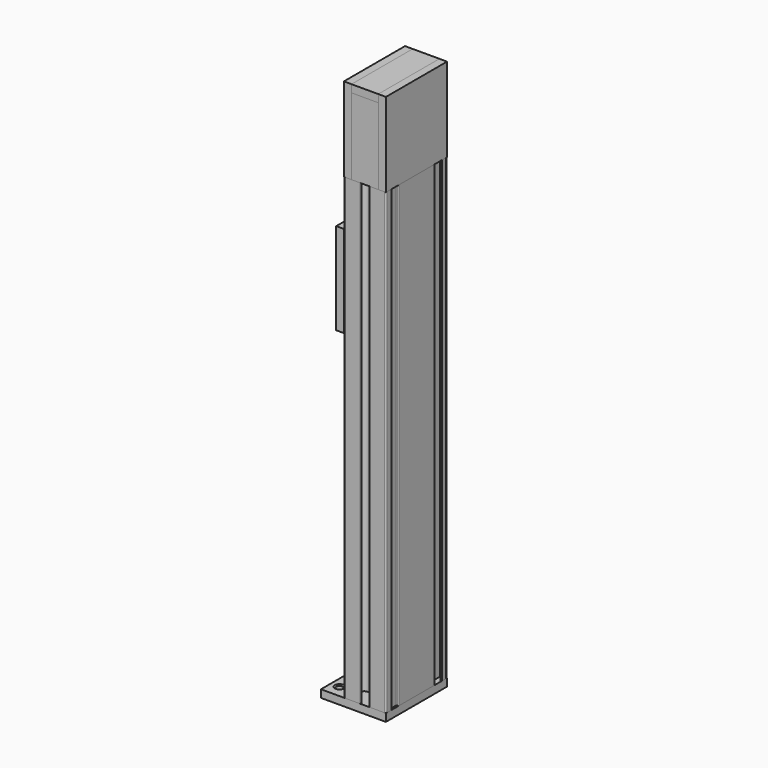
from build123d import *

# Parameters (mm, degrees)
F1_DEPTH        = 600
F2_W            = 100
F2_H            = 110
F3_DEPTH        = 10
F4_W            = 100
F4_H            = 110
F5_DEPTH        = 10
F6_W            = 100
F6_H            = 10
F7_DEPTH        = 35
F8_W            = 35
F8_H            = 100
F9_DEPTH        = 10
F10_W           = 35
F10_H           = 100
F11_DEPTH       = 10
F12_W           = 85
F12_H           = 100
F13_DEPTH       = 10
F15_D           = 9
F15_CSINK_D     = 12
F15_CSINK_ANGLE = 90
F16_W           = 100
F16_H           = 120
F17_DEPTH       = 10
F19_D           = 9
F19_CSINK_D     = 11
F19_CSINK_ANGLE = 90
F21_DEPTH       = 65.001


with BuildPart() as f1:
    # F0 (on Top) → F1 (new body)
    with BuildSketch(Plane.XY):
        with BuildLine():
            Line((8.33733906, -48), (6.5, -48))
            ThreePointArc((6.5, -48), (5.5, -49), (6.5, -50))
            Line((6.5, -50), (25.5, -50))
            ThreePointArc((25.5, -50), (26.9142135624, -49.4142135624), (27.5, -48))
            Line((27.5, -48), (27.5, -41.5))
            ThreePointArc((27.5, -41.5), (27.2071067812, -40.7928932188), (26.5, -40.5))
            Line((26.5, -40.5), (25.30947502, -40.5))
            ThreePointArc((25.30947502, -40.5), (24.9559216294, -40.3535533906), (24.80947502, -40))
            Line((24.80947502, -40), (24.80947502, -30))
            ThreePointArc((24.80947502, -30), (24.9559216294, -29.6464466094), (25.30947502, -29.5))
            Line((25.30947502, -29.5), (26.5, -29.5))
            ThreePointArc((26.5, -29.5), (27.2071067812, -29.2071067812), (27.5, -28.5))
            Line((27.5, -28.5), (27.5, 29))
            ThreePointArc((27.5, 29), (26.5, 30), (25.5, 29))
            Line((25.5, 29), (25.5, 24))
            ThreePointArc((25.5, 24), (25.3535533906, 23.6464466094), (25, 23.5))
            Line((25, 23.5), (20.5, 23.5))
            ThreePointArc((20.5, 23.5), (20.1464466094, 23.6464466094), (20, 24))
            Line((20, 24), (20, 47.5))
            ThreePointArc((20, 47.5), (20.1464466094, 47.8535533906), (20.5, 48))
            Line((20.5, 48), (25, 48))
            ThreePointArc((25, 48), (25.3535533906, 47.8535533906), (25.5, 47.5))
            Line((25.5, 47.5), (25.5, 42))
            ThreePointArc((25.5, 42), (26.5, 41), (27.5, 42))
            Line((27.5, 42), (27.5, 48))
            ThreePointArc((27.5, 48), (26.9142135624, 49.4142135624), (25.5, 50))
            Line((25.5, 50), (7, 50))
            ThreePointArc((7, 50), (6, 49), (7, 48))
            Line((7, 48), (17.5, 48))
            ThreePointArc((17.5, 48), (17.8535533906, 47.8535533906), (18, 47.5))
            Line((18, 47.5), (18, 40.5))
            ThreePointArc((18, 40.5), (17.8535533906, 40.1464466094), (17.5, 40))
            Line((17.5, 40), (-17.5, 40))
            ThreePointArc((-17.5, 40), (-17.8535533906, 40.1464466094), (-18, 40.5))
            Line((-18, 40.5), (-18, 47.5))
            ThreePointArc((-18, 47.5), (-17.8535533906, 47.8535533906), (-17.5, 48))
            Line((-17.5, 48), (-7, 48))
            ThreePointArc((-7, 48), (-6, 49), (-7, 50))
            Line((-7, 50), (-25.5, 50))
            ThreePointArc((-25.5, 50), (-26.9142135624, 49.4142135624), (-27.5, 48))
            Line((-27.5, 48), (-27.5, 42))
            ThreePointArc((-27.5, 42), (-26.5, 41), (-25.5, 42))
            Line((-25.5, 42), (-25.5, 47.5))
            ThreePointArc((-25.5, 47.5), (-25.3535533906, 47.8535533906), (-25, 48))
            Line((-25, 48), (-20.5, 48))
            ThreePointArc((-20.5, 48), (-20.1464466094, 47.8535533906), (-20, 47.5))
            Line((-20, 47.5), (-20, 24))
            ThreePointArc((-20, 24), (-20.1464466094, 23.6464466094), (-20.5, 23.5))
            Line((-20.5, 23.5), (-25, 23.5))
            ThreePointArc((-25, 23.5), (-25.3535533906, 23.6464466094), (-25.5, 24))
            Line((-25.5, 24), (-25.5, 29))
            ThreePointArc((-25.5, 29), (-26.5, 30), (-27.5, 29))
            Line((-27.5, 29), (-27.5, -28.5))
            ThreePointArc((-27.5, -28.5), (-27.2071067812, -29.2071067812), (-26.5, -29.5))
            Line((-26.5, -29.5), (-25.30947502, -29.5))
            ThreePointArc((-25.30947502, -29.5), (-24.9559216294, -29.6464466094), (-24.80947502, -30))
            Line((-24.80947502, -30), (-24.80947502, -40))
            ThreePointArc((-24.80947502, -40), (-24.9559216294, -40.3535533906), (-25.30947502, -40.5))
            Line((-25.30947502, -40.5), (-26.5, -40.5))
            ThreePointArc((-26.5, -40.5), (-27.2071067812, -40.7928932188), (-27.5, -41.5))
            Line((-27.5, -41.5), (-27.5, -48))
            ThreePointArc((-27.5, -48), (-26.9142135624, -49.4142135624), (-25.5, -50))
            Line((-25.5, -50), (-6.5, -50))
            ThreePointArc((-6.5, -50), (-5.5, -49), (-6.5, -48))
            Line((-6.5, -48), (-8.33733906, -48))
            ThreePointArc((-8.33733906, -48), (-8.6908924506, -47.8535533906), (-8.83733906, -47.5))
            Line((-8.83733906, -47.5), (-8.83733906, -46))
            ThreePointArc((-8.83733906, -46), (-8.9837856694, -45.6464466094), (-9.33733906, -45.5))
            Line((-9.33733906, -45.5), (-11.8095842402, -45.5))
            ThreePointArc((-11.8095842402, -45.5), (-12.0057003753, -45.5400668945), (-12.1703854525, -45.6538461538))
            ThreePointArc((-12.1703854525, -45.6538461538), (-17.9864641346, -47.3129531545), (-22.2921545673, -43.0655495741))
            ThreePointArc((-22.2921545673, -43.0655495741), (-22.3051259928, -43.0008907051), (-22.30947502, -42.9350871095))
            Line((-22.30947502, -42.9350871095), (-22.30947502, -29.0649128904))
            ThreePointArc((-22.30947502, -29.0649128904), (-22.3051259928, -28.9991092949), (-22.2921545673, -28.934450426))
            ThreePointArc((-22.2921545673, -28.934450426), (-18.8105481092, -24.9627292431), (-13.5385137945, -25.2818011292))
            ThreePointArc((-13.5385137945, -25.2818011292), (-12.4221432577, -26.0444644798), (-11.0970213481, -26.3127749093))
            Line((-11.0970213481, -26.3127749093), (-9.33733906, -26.3127749093))
            ThreePointArc((-9.33733906, -26.3127749093), (-8.9837856694, -26.1663282999), (-8.83733906, -25.8127749093))
            Line((-8.83733906, -25.8127749093), (-8.83733906, -21.1))
            ThreePointArc((-8.83733906, -21.1), (-8.3687099099, -19.9686291501), (-7.23733906, -19.5))
            Line((-7.23733906, -19.5), (7.23733906, -19.5))
            ThreePointArc((7.23733906, -19.5), (8.3687099099, -19.9686291501), (8.83733906, -21.1))
            Line((8.83733906, -21.1), (8.83733906, -25.8127749093))
            ThreePointArc((8.83733906, -25.8127749093), (8.9837856694, -26.1663282999), (9.33733906, -26.3127749093))
            Line((9.33733906, -26.3127749093), (11.0970213482, -26.3127749093))
            ThreePointArc((11.0970213482, -26.3127749093), (12.4221432577, -26.0444644798), (13.5385137946, -25.2818011292))
            ThreePointArc((13.5385137946, -25.2818011292), (18.8105481092, -24.9627292431), (22.2921545673, -28.9344504259))
            ThreePointArc((22.2921545673, -28.9344504259), (22.3051259928, -28.9991092949), (22.30947502, -29.0649128904))
            Line((22.30947502, -29.0649128904), (22.30947502, -42.9350871095))
            ThreePointArc((22.30947502, -42.9350871095), (22.3051259928, -43.0008907051), (22.2921545673, -43.0655495741))
            ThreePointArc((22.2921545673, -43.0655495741), (17.9864641346, -47.3129531545), (12.1703854525, -45.6538461538))
            ThreePointArc((12.1703854525, -45.6538461538), (12.0057003753, -45.5400668945), (11.8095842402, -45.5))
            Line((11.8095842402, -45.5), (9.33733906, -45.5))
            ThreePointArc((9.33733906, -45.5), (8.9837856694, -45.6464466094), (8.83733906, -46))
            Line((8.83733906, -46), (8.83733906, -47.5))
            ThreePointArc((8.83733906, -47.5), (8.6908924506, -47.8535533906), (8.33733906, -48))
        make_face()
        with BuildLine():
            Line((25.5, 14.6098564162), (25.5, -14.1098564162))
            ThreePointArc((25.5, -14.1098564162), (25.2937023297, -14.5145031034), (24.8450442339, -14.5852391152))
            ThreePointArc((24.8450442339, -14.5852391152), (23.1777547131, -15.1146259293), (23.1458153918, -16.8636498356))
            ThreePointArc((23.1458153918, -16.8636498356), (21.5, -20), (19.8541846082, -16.8636498356))
            ThreePointArc((19.8541846082, -16.8636498356), (19.4720856876, -14.7770256685), (17.3854615204, -15.1591245891))
            ThreePointArc((17.3854615204, -15.1591245891), (16.5045669812, -18.2136561594), (17.6430539208, -21.1818181818))
            ThreePointArc((17.6430539208, -21.1818181818), (17.7096263297, -21.7132007164), (17.2573593129, -22))
            Line((17.2573593129, -22), (11.83733906, -22))
            ThreePointArc((11.83733906, -22), (11.4837856694, -21.8535533906), (11.33733906, -21.5))
            Line((11.33733906, -21.5), (11.33733906, -21.1))
            ThreePointArc((11.33733906, -21.1), (10.1364768629, -18.2008621971), (7.23733906, -17))
            Line((7.23733906, -17), (-7.23733906, -17))
            ThreePointArc((-7.23733906, -17), (-10.1364768629, -18.2008621971), (-11.33733906, -21.1))
            Line((-11.33733906, -21.1), (-11.33733906, -21.5))
            ThreePointArc((-11.33733906, -21.5), (-11.4837856694, -21.8535533906), (-11.83733906, -22))
            Line((-11.83733906, -22), (-17.2573593129, -22))
            ThreePointArc((-17.2573593129, -22), (-17.7096263297, -21.7132007164), (-17.6430539208, -21.1818181818))
            ThreePointArc((-17.6430539208, -21.1818181818), (-16.5045669812, -18.2136561594), (-17.3854615204, -15.1591245891))
            ThreePointArc((-17.3854615204, -15.1591245891), (-19.4720856876, -14.7770256685), (-19.8541846082, -16.8636498356))
            ThreePointArc((-19.8541846082, -16.8636498356), (-21.5, -20), (-23.1458153918, -16.8636498356))
            ThreePointArc((-23.1458153918, -16.8636498356), (-23.1777547131, -15.1146259293), (-24.8450442339, -14.5852391152))
            ThreePointArc((-24.8450442339, -14.5852391152), (-25.2937023297, -14.5145031034), (-25.5, -14.1098564162))
            Line((-25.5, -14.1098564162), (-25.5, 14.6098564162))
            ThreePointArc((-25.5, 14.6098564162), (-25.2937023297, 15.0145031034), (-24.8450442339, 15.0852391152))
            ThreePointArc((-24.8450442339, 15.0852391152), (-23.1777547131, 15.6146259293), (-23.1458153918, 17.3636498356))
            ThreePointArc((-23.1458153918, 17.3636498356), (-21.5, 20.5), (-19.8541846082, 17.3636498356))
            ThreePointArc((-19.8541846082, 17.3636498356), (-19.4720856876, 15.2770256685), (-17.3854615204, 15.6591245891))
            ThreePointArc((-17.3854615204, 15.6591245891), (-16.514462151, 18.8800162584), (-17.8635792315, 21.9316823854))
            ThreePointArc((-17.8635792315, 21.9316823854), (-17.9646454387, 22.0902903218), (-18, 22.2750087852))
            Line((-18, 22.2750087852), (-18, 36.5))
            ThreePointArc((-18, 36.5), (-17.7071067812, 37.2071067812), (-17, 37.5))
            Line((-17, 37.5), (17, 37.5))
            ThreePointArc((17, 37.5), (17.7071067812, 37.2071067812), (18, 36.5))
            Line((18, 36.5), (18, 22.2750087852))
            ThreePointArc((18, 22.2750087852), (17.9646454387, 22.0902903218), (17.8635792315, 21.9316823854))
            ThreePointArc((17.8635792315, 21.9316823854), (16.514462151, 18.8800162584), (17.3854615204, 15.6591245891))
            ThreePointArc((17.3854615204, 15.6591245891), (19.4720856876, 15.2770256685), (19.8541846082, 17.3636498356))
            ThreePointArc((19.8541846082, 17.3636498356), (19.6774992234, 19.3237056022), (21.2654667699, 20.4862009375))
            ThreePointArc((21.2654667699, 20.4862009375), (22.3229466011, 17.3003700971), (24.8450442339, 15.0852391152))
            ThreePointArc((24.8450442339, 15.0852391152), (25.2937023297, 15.0145031034), (25.5, 14.6098564162))
        make_face(mode=Mode.SUBTRACT)
    extrude(amount=-F1_DEPTH)


with BuildPart() as f3:
    # F2 (on face) → F3 (new body)
    with BuildSketch(Plane.YZ.offset(27.5)):
        with Locations((0, 55)):
            Rectangle(F2_W, F2_H)
    extrude(amount=-F3_DEPTH)


with BuildPart() as f5:
    # F4 (on face) → F5 (new body)
    with BuildSketch(Plane(origin=(-27.5, 0, 0), x_dir=(0, -1, 0), z_dir=(-1, 0, 0))):
        with Locations((0, 55)):
            Rectangle(F4_W, F4_H)
    extrude(amount=-F5_DEPTH)


with BuildPart() as f7:
    # F6 (on face) → F7 (new body, through all)
    with BuildSketch(Plane(origin=(17.5, 0, 0), x_dir=(0, -1, 0), z_dir=(-1, 0, 0))):
        with Locations((0, 105)):
            Rectangle(F6_W, F6_H)
    extrude(amount=F7_DEPTH)


with BuildPart() as f9:
    # F8 (on face) → F9 (new body)
    with BuildSketch(Plane.XZ.offset(50)):
        with Locations((0, 50)):
            Rectangle(F8_W, F8_H)
    extrude(amount=-F9_DEPTH)


with BuildPart() as f11:
    # F10 (on face) → F11 (new body)
    with BuildSketch(Plane(origin=(0, 50, 0), x_dir=(-1, 0, 0), z_dir=(0, 1, 0))):
        with Locations((0, 50)):
            Rectangle(F10_W, F10_H)
    extrude(amount=-F11_DEPTH)


with BuildPart() as f13:
    # F12 (on face) → F13 (new body)
    with BuildSketch(Plane(origin=(0, 0, -600), x_dir=(1, 0, 0), z_dir=(0, 0, -1))):
        with Locations((-15, 0)):
            Rectangle(F12_W, F12_H)
    extrude(amount=F13_DEPTH)

    # F15 (through all)
    with Locations(Plane.XY.offset(-600)):
        with Locations((-46.1519472301, 34.3138426542), (-46.1519472301, -33.9523144066)):
            CounterSinkHole(F15_D / 2, F15_CSINK_D / 2, counter_sink_angle=F15_CSINK_ANGLE)


with BuildPart() as f17:
    # F16 (on face) → F17 (new body)
    with BuildSketch(Plane(origin=(-27.5, 0, 0), x_dir=(0, -1, 0), z_dir=(-1, 0, 0))):
        with Locations((0, -120)):
            Rectangle(F16_W, F16_H)
    extrude(amount=F17_DEPTH)

    # F19 (through all)
    with Locations(Plane(origin=(-37.5, 0, 0), x_dir=(0, -1, 0), z_dir=(-1, 0, 0))):
        with Locations((-35.5, -70), (-35.5, -170)):
            CounterSinkHole(F19_D / 2, F19_CSINK_D / 2, counter_sink_angle=F19_CSINK_ANGLE)

    # F20 (on face) → F21 (cut, through all)
    with BuildSketch(Plane(origin=(-37.5, 0, 0), x_dir=(0, -1, 0), z_dir=(-1, 0, 0))):
        with BuildLine():
            Line((-40, -146.9999998083), (0, -146.9999998083))
            ThreePointArc((0, -146.9999998083), (26.1629509039, -136.1629507122), (37, -109.9999998083))
            Line((37, -109.9999998083), (37, -100.0000001917))
            ThreePointArc((37, -100.0000001917), (30, -93.0000001917), (23, -100.0000001917))
            Line((23, -100.0000001917), (23, -109.9999998083))
            ThreePointArc((23, -109.9999998083), (16.2634559673, -126.2634557756), (0, -132.9999998083))
            Line((0, -132.9999998083), (-40, -132.9999998083))
            ThreePointArc((-40, -132.9999998083), (-47, -139.9999998083), (-40, -146.9999998083))
        make_face()
    extrude(amount=-F21_DEPTH, mode=Mode.SUBTRACT)


solid = Compound([f1.part, f3.part, f5.part, f7.part, f9.part, f11.part, f13.part, f17.part])
